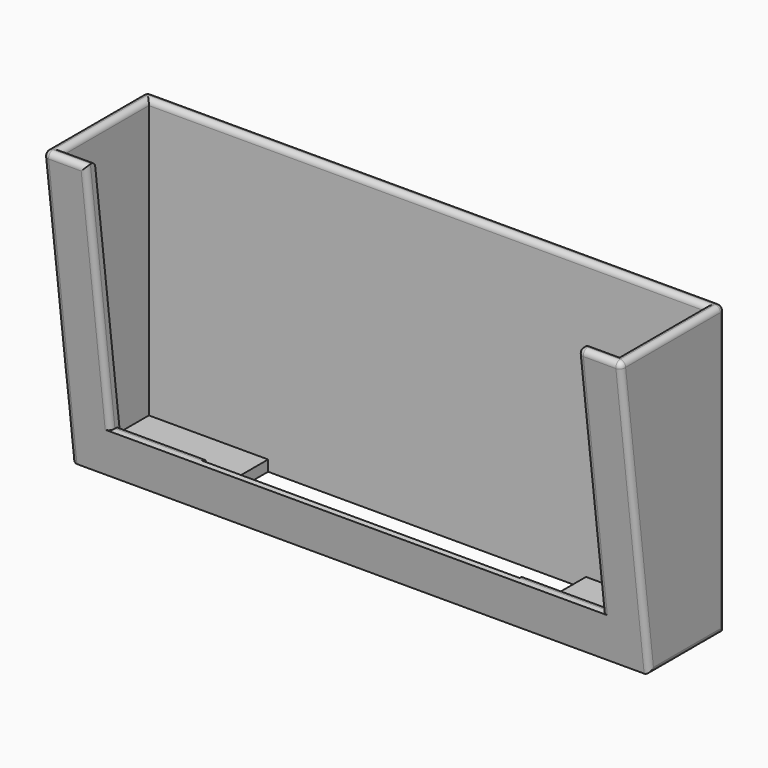
from build123d import *

# Parameters (mm, degrees)
F0_W     = 80
F0_H     = 13
F2_W     = 80
F2_H     = 18
F4_T     = -1.5
F5_W     = 68
F5_H     = 34.3112887415
F6_DEPTH = 2.7
F7_W     = 44
F7_H     = 11.5
F8_DEPTH = 25
F9_R     = 0.74999


# Not quite as in the source:
# - a fillet or chamfer is up to 0.001 mm smaller than in the source, because OpenCascade refuses the exact size


with BuildPart() as f3:
    # F0 (on Top) → F3 section 0
    with BuildSketch(Plane.XY):
        with Locations((40, -6.5)):
            Rectangle(F0_W, F0_H)
    # F2 (on offset) → F3 section 1
    with BuildSketch(Plane.XY.offset(40)):
        with Locations((40, -9)):
            Rectangle(F2_W, F2_H)
    loft()

    # F4
    f4_openings = [f3.faces().sort_by_distance(p)[0] for p in [
        (40, -9, 40),
    ]]
    offset(amount=F4_T, openings=f4_openings)

    # F5 (on face) → F6 (cut)
    with BuildSketch(Plane(origin=(0, -12.8, -1.6), x_dir=(1, 0, 0), z_dir=(0, -0.9922778767, -0.1240347346))):
        with Locations((40, 24.7680959204)):
            Rectangle(F5_W, F5_H)
    extrude(amount=-F6_DEPTH, mode=Mode.SUBTRACT)

    # F7 (on face) → F8 (cut)
    with BuildSketch(Plane(origin=(0, 0, 0), x_dir=(1, 0, 0), z_dir=(0, 0, -1))):
        with Locations((40, 7.25)):
            Rectangle(F7_W, F7_H)
    extrude(amount=-F8_DEPTH, mode=Mode.SUBTRACT)

    # F9 (radius 0.75 in the source; OpenCascade refuses exactly that, so slightly less here)
    f9_edges = [f3.edges().sort_by_distance(p)[0] for p in [
        (80, -15.5, 20),
        (80, -6.5, 0),
        (80, 0, 20),
        (0, -15.5, 20),
        (0, 0, 20),
        (0, -6.5, 0),
        (6, -15.872104, 22.976834),
        (74, -15.872104, 22.976834),
        (3, -18, 40),
        (77, -18, 40),
        (80, -9, 40),
        (74, -17.244163, 40),
        (0, -9, 40),
        (40, 0, 40),
        (3.75, -16.488327, 40),
        (1.5, -8.994163, 40),
        (40, -1.5, 40),
        (78.5, -8.994163, 40),
        (76.25, -16.488327, 40),
        (12, -12.255792, 6.139719),
        (68, -12.255792, 6.139719),
    ]]
    fillet(f9_edges, radius=F9_R)


solid = f3.part
